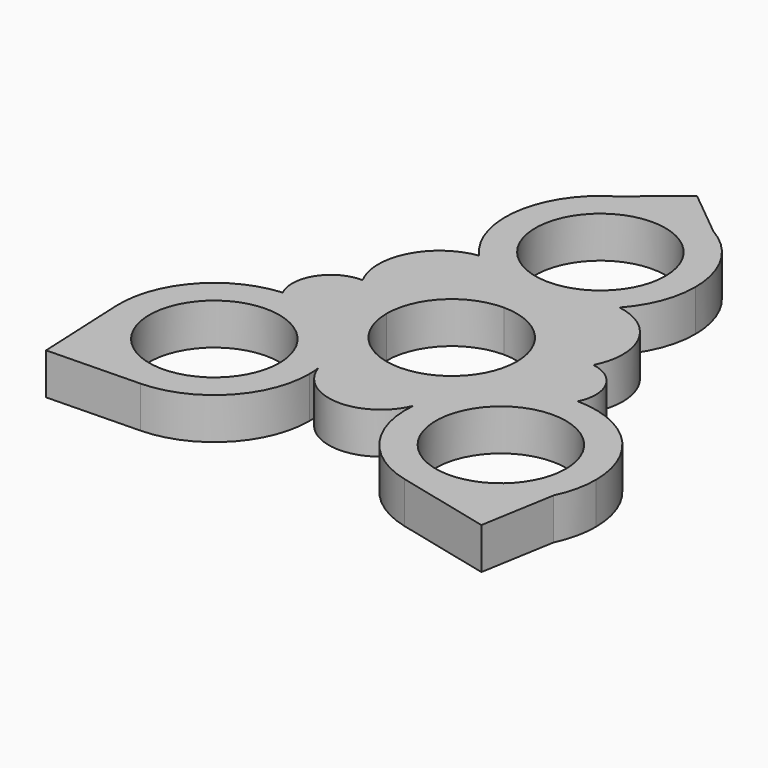
from build123d import *

# Parameters (mm, degrees)
F0_R     = 11.049
F1_DEPTH = 7.0358


with BuildPart() as f1:
    # F0 (on Top) → F1 (new body)
    with BuildSketch(Plane.XY):
        with BuildLine():
            ThreePointArc((15.3606223584, -6.5915638429), (14.0515764921, -2.7419023957), (11.049, 0))
            ThreePointArc((11.049, 0), (7.8128228253, -7.8128228253), (0, -11.049))
            ThreePointArc((0, -11.049), (3.7722273632, -14.6239373815), (8.9372329685, -15.2006467181))
            ThreePointArc((8.9372329685, -15.2006467181), (11.4112106852, -10.3456815617), (15.3606223584, -6.5915638429))
        make_face()
        with BuildLine():
            ThreePointArc((0, 11.049), (7.8128228253, 7.8128228253), (11.049, 0))
            ThreePointArc((11.049, 0), (16.0517409884, 1.6673539034), (19.5923287649, 5.5752593056))
            ThreePointArc((19.5923287649, 5.5752593056), (19.648285181, 15.0586380241), (11.9809254143, 20.639784613))
            ThreePointArc((11.9809254143, 20.639784613), (7.1318081537, 17.0036295078), (1.2830021666, 15.4139658073))
            ThreePointArc((1.2830021666, 15.4139658073), (0.3997348377, 13.3025456864), (0, 11.049))
        make_face()
        with BuildLine():
            ThreePointArc((19.5923287649, 5.5752593056), (16.0517409884, 1.6673539034), (11.049, 0))
            ThreePointArc((11.049, 0), (14.0515764921, -2.7419023957), (15.3606223584, -6.5915638429))
            ThreePointArc((15.3606223584, -6.5915638429), (19.7194060635, -4.5374863882), (24.4904460645, -3.8626479736))
            ThreePointArc((24.4904460645, -3.8626479736), (24.4551845175, 2.1090263166), (19.5923287649, 5.5752593056))
        make_face()
        with BuildLine():
            ThreePointArc((-1.2878785477, 15.4227450117), (-0.401152017, 13.3073628417), (0, 11.049))
            ThreePointArc((0, 11.049), (0.3997348377, 13.3025456864), (1.2830021666, 15.4139658073))
            ThreePointArc((1.2830021666, 15.4139658073), (-0.0026133903, 15.367050345), (-1.2878785477, 15.4227450117))
        make_face()
        with BuildLine():
            ThreePointArc((-11.049, 0), (-7.8128228253, 7.8128228253), (0, 11.049))
            ThreePointArc((0, 11.049), (-0.401152017, 13.3073628417), (-1.2878785477, 15.4227450117))
            ThreePointArc((-1.2878785477, 15.4227450117), (-7.0848261597, 17.032079869), (-11.8887450472, 20.6538092378))
            ThreePointArc((-11.8887450472, 20.6538092378), (-19.6475824124, 15.060028688), (-19.5503933089, 5.4954851872))
            ThreePointArc((-19.5503933089, 5.4954851872), (-16.0139499505, 1.6428086369), (-11.049, 0))
        make_face()
        with BuildLine():
            ThreePointArc((-8.7698737274, -15.7762258045), (-3.5991350923, -14.870419784), (0, -11.049))
            ThreePointArc((0, -11.049), (-7.8128228253, -7.8128228253), (-11.049, 0))
            ThreePointArc((-11.049, 0), (-14.2101099006, -2.5648530064), (-15.7760277941, -6.3223771779))
            ThreePointArc((-15.7760277941, -6.3223771779), (-11.380052467, -10.3875833636), (-8.7698737274, -15.7762258045))
        make_face()
        with BuildLine():
            ThreePointArc((8.9372329685, -15.2006467181), (3.7722273632, -14.6239373815), (0, -11.049))
            ThreePointArc((0, -11.049), (-3.5991350923, -14.870419784), (-8.7698737274, -15.7762258045))
            ThreePointArc((-8.7698737274, -15.7762258045), (-8.5203506621, -16.839417556), (-8.3433460468, -17.9170574897))
            ThreePointArc((-8.3433460468, -17.9170574897), (-0.2261466235, -23.9881077254), (8.2807318523, -18.4763388586))
            ThreePointArc((8.2807318523, -18.4763388586), (8.523941199, -16.8214491689), (8.9372329685, -15.2006467181))
        make_face()
        with BuildLine():
            ThreePointArc((8.9372329685, -15.2006467181), (13.7625460617, -12.1000545802), (15.3606223584, -6.5915638429))
            ThreePointArc((15.3606223584, -6.5915638429), (11.4112106852, -10.3456815617), (8.9372329685, -15.2006467181))
        make_face()
        with BuildLine():
            ThreePointArc((24.4904460645, -3.8626479736), (20.5132557556, -7.1933790888), (15.3606223584, -6.5915638429))
            ThreePointArc((15.3606223584, -6.5915638429), (13.7625460617, -12.1000545802), (8.9372329685, -15.2006467181))
            ThreePointArc((8.9372329685, -15.2006467181), (8.7646746362, -16.8696960014), (8.2807318523, -18.4763388586))
            ThreePointArc((8.2807318523, -18.4763388586), (11.2032111335, -29.3509460419), (20.5279860839, -35.6633575195))
            ThreePointArc((20.5279860839, -35.6633575195), (31.2506997753, -34.5637006191), (38.8862682367, -26.9555517986))
            ThreePointArc((38.8862682367, -26.9555517986), (40.0671958518, -23.5618596089), (40.4674604904, -19.9909318682))
            ThreePointArc((40.4674604904, -19.9909318682), (35.7969947842, -8.6398687974), (24.4904460645, -3.8626479736))
        make_face()
        with Locations((24.3384604904, -19.9909318682)):
            Circle(F0_R, mode=Mode.SUBTRACT)
        with BuildLine():
            ThreePointArc((24.4904460645, -3.8626479736), (19.7194060635, -4.5374863882), (15.3606223584, -6.5915638429))
            ThreePointArc((15.3606223584, -6.5915638429), (20.5132557556, -7.1933790888), (24.4904460645, -3.8626479736))
        make_face()
        with BuildLine():
            ThreePointArc((-15.7760277941, -6.3223771779), (-14.2101099006, -2.5648530064), (-11.049, 0))
            ThreePointArc((-11.049, 0), (-16.0139499505, 1.6428086369), (-19.5503933089, 5.4954851872))
            ThreePointArc((-19.5503933089, 5.4954851872), (-25.2039351491, 2.4834340402), (-25.5915562379, -3.9106833611))
            ThreePointArc((-25.5915562379, -3.9106833611), (-20.4899973654, -4.3277912963), (-15.7760277941, -6.3223771779))
        make_face()
        with BuildLine():
            ThreePointArc((2.1504403371, 16.730865023), (1.6917102547, 16.0888900954), (1.2830021666, 15.4139658073))
            ThreePointArc((1.2830021666, 15.4139658073), (7.1318081537, 17.0036295078), (11.9809254143, 20.639784613))
            ThreePointArc((11.9809254143, 20.639784613), (6.5311461577, 20.0296234429), (2.1504403371, 16.730865023))
        make_face()
        with BuildLine():
            ThreePointArc((-1.2878785477, 15.4227450117), (-0.0026133903, 15.367050345), (1.2830021666, 15.4139658073))
            ThreePointArc((1.2830021666, 15.4139658073), (1.6917102547, 16.0888900954), (2.1504403371, 16.730865023))
            ThreePointArc((2.1504403371, 16.730865023), (-0.0310099814, 18.9779969426), (-2.0205494764, 16.5593072242))
            ThreePointArc((-2.0205494764, 16.5593072242), (-1.6357105315, 16.0029541604), (-1.2878785477, 15.4227450117))
        make_face()
        with BuildLine():
            ThreePointArc((-11.8887450472, 20.6538092378), (-7.0848261597, 17.032079869), (-1.2878785477, 15.4227450117))
            ThreePointArc((-1.2878785477, 15.4227450117), (-1.6357105315, 16.0029541604), (-2.0205494764, 16.5593072242))
            ThreePointArc((-2.0205494764, 16.5593072242), (-6.3882732082, 19.9715813543), (-11.8887450472, 20.6538092378))
        make_face()
        with BuildLine():
            ThreePointArc((8.2807318523, -18.4763388586), (8.7646746362, -16.8696960014), (8.9372329685, -15.2006467181))
            ThreePointArc((8.9372329685, -15.2006467181), (8.523941199, -16.8214491689), (8.2807318523, -18.4763388586))
        make_face()
        with BuildLine():
            ThreePointArc((-15.7760277941, -6.3223771779), (-14.2311309419, -12.5004895292), (-8.7698737274, -15.7762258045))
            ThreePointArc((-8.7698737274, -15.7762258045), (-11.380052467, -10.3875833636), (-15.7760277941, -6.3223771779))
        make_face()
        with BuildLine():
            ThreePointArc((-8.3433460468, -17.9170574897), (-8.6227516064, -16.8598193641), (-8.7698737274, -15.7762258045))
            ThreePointArc((-8.7698737274, -15.7762258045), (-14.2311309419, -12.5004895292), (-15.7760277941, -6.3223771779))
            ThreePointArc((-15.7760277941, -6.3223771779), (-21.2515182716, -7.4271607367), (-25.5915562379, -3.9106833611))
            ThreePointArc((-25.5915562379, -3.9106833611), (-36.4277245579, -9.3141188931), (-40.450284213, -20.7350940367))
            ThreePointArc((-40.450284213, -20.7350940367), (-35.3407505097, -31.7847546298), (-23.963299648, -36.1155681538))
            ThreePointArc((-23.963299648, -36.1155681538), (-12.8016582856, -31.2624373527), (-8.2094604904, -19.9909318682))
            ThreePointArc((-8.2094604904, -19.9909318682), (-8.2429666822, -18.9518360737), (-8.3433460468, -17.9170574897))
        make_face()
        with Locations((-24.3384604904, -19.9909318682)):
            Circle(F0_R, mode=Mode.SUBTRACT)
        with BuildLine():
            ThreePointArc((-8.3433460468, -17.9170574897), (-8.5203506621, -16.839417556), (-8.7698737274, -15.7762258045))
            ThreePointArc((-8.7698737274, -15.7762258045), (-8.6227516064, -16.8598193641), (-8.3433460468, -17.9170574897))
        make_face()
        with BuildLine():
            ThreePointArc((2.1504403371, 16.730865023), (6.5311461577, 20.0296234429), (11.9809254143, 20.639784613))
            ThreePointArc((11.9809254143, 20.639784613), (15.0947181843, 25.6757116075), (16.1814646071, 31.4959563034))
            ThreePointArc((16.1814646071, 31.4959563034), (14.0032432118, 39.5904246198), (8.0569166098, 45.4985770987))
            ThreePointArc((8.0569166098, 45.4985770987), (-0.1661064271, 47.6234752602), (-8.3285237566, 45.2765105392))
            ThreePointArc((-8.3285237566, 45.2765105392), (-15.9105328531, 33.804062255), (-11.8887450472, 20.6538092378))
            ThreePointArc((-11.8887450472, 20.6538092378), (-6.3882732082, 19.9715813543), (-2.0205494764, 16.5593072242))
            ThreePointArc((-2.0205494764, 16.5593072242), (-0.0310099814, 18.9779969426), (2.1504403371, 16.730865023))
        make_face()
        with Locations((0.0524646071, 31.4959563034)):
            Circle(F0_R, mode=Mode.SUBTRACT)
        with BuildLine():
            ThreePointArc((-25.5915562379, -3.9106833611), (-21.2515182716, -7.4271607367), (-15.7760277941, -6.3223771779))
            ThreePointArc((-15.7760277941, -6.3223771779), (-20.4899973654, -4.3277912963), (-25.5915562379, -3.9106833611))
        make_face()
        with BuildLine():
            Line((0, 52.0859286189), (-8.3285237566, 45.2765105392))
            ThreePointArc((-8.3285237566, 45.2765105392), (-0.1661064271, 47.6234752602), (8.0569166098, 45.4985770987))
            Line((8.0569166098, 45.4985770987), (0, 52.0859286189))
        make_face()
        with BuildLine():
            ThreePointArc((38.8862682367, -26.9555517986), (31.2506997753, -34.5637006191), (20.5279860839, -35.6633575195))
            Line((20.5279860839, -35.6633575195), (36.7174671022, -39.5995448364))
            Line((36.7174671022, -39.5995448364), (38.8862682367, -26.9555517986))
        make_face()
        with BuildLine():
            ThreePointArc((-23.963299648, -36.1155681538), (-35.3407505097, -31.7847546298), (-40.450284213, -20.7350940367))
            Line((-40.450284213, -20.7350940367), (-39.7229656538, -36.4822374832))
            Line((-39.7229656538, -36.4822374832), (-23.963299648, -36.1155681538))
        make_face()
    extrude(amount=F1_DEPTH)


solid = f1.part
